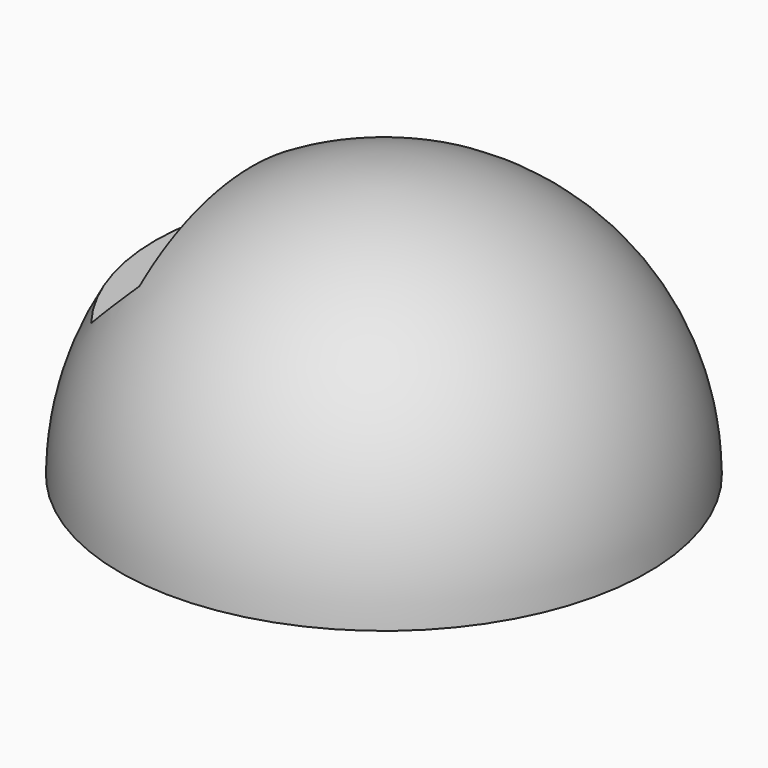
from build123d import *
from build123d import SkipClean  # not in build123d's __all__

# Parameters (mm, degrees)
F3_DEPTH = 127


with BuildPart() as f1:
    # F0 (on Front) → F1 (revolve)
    with BuildSketch(Plane.XZ):
        with BuildLine():
            Line((-63.5, -63.5), (-50.8, -63.5))
            ThreePointArc((-50.8, -63.5), (-17.3223050896, 17.3223050896), (63.5, 50.8))
            Line((63.5, 50.8), (63.5, 63.5))
            ThreePointArc((63.5, 63.5), (-26.3025612107, 26.3025612107), (-63.5, -63.5))
        make_face()
    revolve(axis=Axis((63.5, 0, 0), (0, 0, -1)))

    # F2 (on Front) → F3 (cut, symmetric)
    with BuildSketch(Plane.XZ):
        with BuildLine():
            Line((-46.4852262806, 0), (0, 46.4852262806))
            ThreePointArc((0, 46.4852262806), (-26.3025612107, 26.3025612107), (-46.4852262806, 0))
        make_face()
        Polygon((0, 23.2426131403), (0, 46.4852262806), (-46.4852262806, 0), (-23.2426131403, 0), align=None)
    with SkipClean():  # cleaning this boolean's faces spoils the solid; the shape is the same uncleaned
        extrude(amount=F3_DEPTH, both=True, mode=Mode.SUBTRACT)


with BuildPart() as f1b:
    # F0 (on Front) → F1, piece 2 (revolve)
    with BuildSketch(Plane.XZ):
        with BuildLine():
            Line((-38.1, -63.5), (63.5, -63.5))
            Line((63.5, -63.5), (63.5, 38.1))
            ThreePointArc((63.5, 38.1), (-8.3420489686, 8.3420489686), (-38.1, -63.5))
        make_face()
    revolve(axis=Axis((63.5, 0, 0), (0, 0, -1)))


solid = Compound([f1.part, f1b.part])
